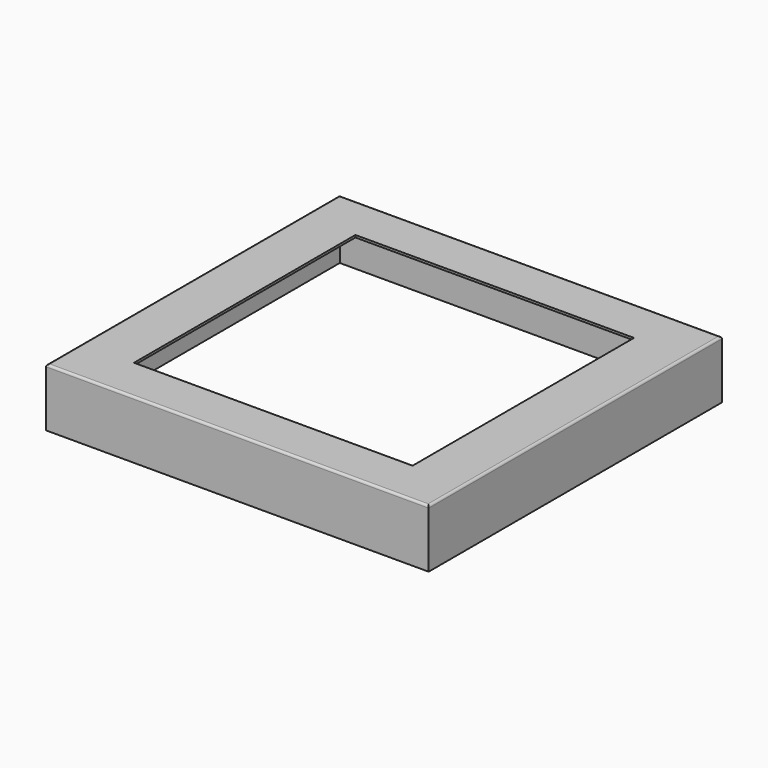
from build123d import *

# Parameters (mm, degrees)
F0_W     = 86.8310853839
F0_H     = 83.1971988082
F1_DEPTH = 13.208
F2_R     = 0.508
F3_T     = 0.508
F4_W     = 63.2273703814
F4_H     = 62.8109127283
F5_DEPTH = 17.272


# Not quite as in the source:
# - a shell that OpenCascade refuses in one call is made with other operations: the cavity is built on its own and cut out


with BuildPart() as f1:
    # F0 (on Top) → F1 (new body)
    with BuildSketch(Plane.XY):
        Rectangle(F0_W, F0_H)
    extrude(amount=F1_DEPTH)

    # F2
    f2_edges = [f1.edges().sort_by_distance(p)[0] for p in [
        (0, -41.598599, 13.208),
        (-43.415543, 0, 13.208),
        (0, 41.598599, 13.208),
        (43.415543, 0, 13.208),
    ]]
    fillet(f2_edges, radius=F2_R)

    # F3: shell of thickness 0.508, made by hand


with BuildPart() as f3_core1:
    # F3_t2: copy of F1
    add(f1.part)

    # the walls: a layer under each face that stays
    f3_faces = [f3_core1.faces().sort_by_distance(p)[0] for p in [
        (0, -41.5985994041, 6.35),
        (-43.4155426919, 0, 6.35),
        (43.4155426919, 0, 6.35),
        (0, 41.5985994041, 6.35),
        (0, 0, 13.208),
    ]]
    thicken(f3_faces, amount=-F3_T, mode=Mode.SUBTRACT)


with BuildPart() as f1_1:
    add(f1.part)

    # what is left inside the walls is the cavity
    f3_cavity = [f3_core1.part.solids().sort_by_distance(p)[0] for p in [
        (0, -13.696866, 12.69492),
    ]]
    add(f3_cavity, mode=Mode.SUBTRACT)

    # F4 (on face) → F5 (cut)
    with BuildSketch(Plane.XY.offset(13.208)):
        Rectangle(F4_W, F4_H)
    extrude(amount=-F5_DEPTH, mode=Mode.SUBTRACT)


solid = f1_1.part
